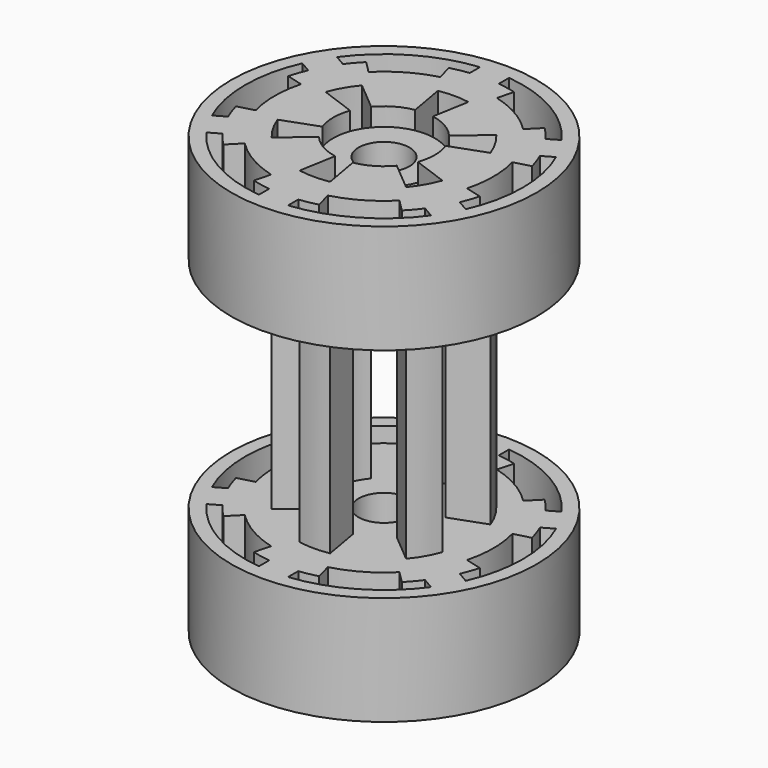
from build123d import *

# Parameters (mm, degrees)
F0_R            = 26.67
F0_R_2          = 4.445
F1_DEPTH        = 19.05
F3_DEPTH        = 19.051
F3_COPIES_COUNT = 6
F6_DEPTH        = 19.051
F6_COPIES_COUNT = 6
F7_R            = 8.8739289646
F8_DEPTH        = 3.175
F10_DEPTH       = 38.1
F11_COUNT       = 6


# Not quite as in the source:
# - a pattern or mirror of a feature is missing from the dataset's text; its kind, count and spacing are read off the source's solid


with BuildPart() as f1:
    # F0 (on Top) → F1 (new body)
    with BuildSketch(Plane.XY):
        Circle(F0_R)
        Circle(F0_R_2, mode=Mode.SUBTRACT)
    extrude(amount=F1_DEPTH)

    # F2 (on face) → F3 (cut, through all)
    with BuildSketch(Plane.XY.offset(19.05)):
        with BuildLine():
            Line((-2.54, 21.8982800173), (-2.54, 24.1282167909))
            ThreePointArc((-2.54, 24.1282167909), (-12.1307712606, 21.0111121583), (-19.6256486889, 14.263812921))
            Line((-19.6256486889, 14.263812921), (-17.6944667941, 13.1488445342))
            ThreePointArc((-17.6944667941, 13.1488445342), (-16.6859897065, 14.4070821205), (-15.5882370349, 15.5882370349))
            Line((-15.5882370349, 15.5882370349), (-13.512959721, 13.512959721))
            ThreePointArc((-13.512959721, 13.512959721), (-9.5551054526, 16.5499281156), (-4.9460865382, 18.4590462592))
            Line((-4.9460865382, 18.4590462592), (-5.705690755, 21.2939277899))
            ThreePointArc((-5.705690755, 21.2939277899), (-4.1339042575, 21.6540320334), (-2.54, 21.8982800173))
        make_face()
    f3 = extrude(amount=-F3_DEPTH, mode=Mode.SUBTRACT)

    # F3_copies: F3 ×6 about axis
    f3_copies_axis = Axis((0, 0, 0), (0, 0, 1))
    for i in range(1, F3_COPIES_COUNT):
        add(f3.rotate(f3_copies_axis, i * 360 / F3_COPIES_COUNT), mode=Mode.SUBTRACT)

    # F5 (on face) → F6 (cut, through all)
    with BuildSketch(Plane.XY.offset(19.05)):
        with BuildLine():
            ThreePointArc((2.6620689543, 15.0973432633), (0, 15.3302441183), (-2.6620689543, 15.0973432633))
            Line((-2.6620689543, 15.0973432633), (-1.5409415934, 8.739114044))
            ThreePointArc((-1.5409415934, 8.739114044), (0, 8.8739289646), (1.5409415934, 8.739114044))
            Line((1.5409415934, 8.739114044), (2.6620689543, 15.0973432633))
        make_face()
    f6 = extrude(amount=-F6_DEPTH, mode=Mode.SUBTRACT)

    # F6_copies: F6 ×6 about axis
    f6_copies_axis = Axis((0, 0, 0), (0, 0, 1))
    for i in range(1, F6_COPIES_COUNT):
        add(f6.rotate(f6_copies_axis, i * 360 / F6_COPIES_COUNT), mode=Mode.SUBTRACT)

    # F7 (on face) → F8 (cut)
    with BuildSketch(Plane.XY.offset(19.05)):
        Circle(F7_R)
    extrude(amount=-F8_DEPTH, mode=Mode.SUBTRACT)


with BuildPart() as f10:
    # F9 (on face) → F10 (new body)
    with BuildSketch(Plane(origin=(0, 0, 0), x_dir=(1, 0, 0), z_dir=(0, 0, -1))):
        with BuildLine():
            Line((-1.5409415934, -8.739114044), (-2.6620689543, -15.0973432633))
            ThreePointArc((-2.6620689543, -15.0973432633), (0, -15.3302441183), (2.6620689543, -15.0973432633))
            Line((2.6620689543, -15.0973432633), (1.5409415934, -8.739114044))
            ThreePointArc((1.5409415934, -8.739114044), (0, -8.8739289646), (-1.5409415934, -8.739114044))
        make_face()
    extrude(amount=F10_DEPTH)


with BuildPart() as f11_1:
    # F11: instance of F10
    add(f10.part.rotate(Axis((0, 0, 32.5610087602), (0, 0, -1)), 1 * 360 / F11_COUNT))


with BuildPart() as f11_2:
    # F11: instance of F10
    add(f10.part.rotate(Axis((0, 0, 32.5610087602), (0, 0, -1)), 2 * 360 / F11_COUNT))


with BuildPart() as f11_3:
    # F11: instance of F10
    add(f10.part.rotate(Axis((0, 0, 32.5610087602), (0, 0, -1)), 3 * 360 / F11_COUNT))


with BuildPart() as f11_4:
    # F11: instance of F10
    add(f10.part.rotate(Axis((0, 0, 32.5610087602), (0, 0, -1)), 4 * 360 / F11_COUNT))


with BuildPart() as f11_5:
    # F11: instance of F10
    add(f10.part.rotate(Axis((0, 0, 32.5610087602), (0, 0, -1)), 5 * 360 / F11_COUNT))


with BuildPart() as f13_1:
    # F13: instance of F1
    add(f1.part.mirror(Plane.XY.offset(-19.05)))


solid = Compound([f1.part, f10.part, f11_1.part, f11_2.part, f11_3.part, f11_4.part, f11_5.part, f13_1.part])
